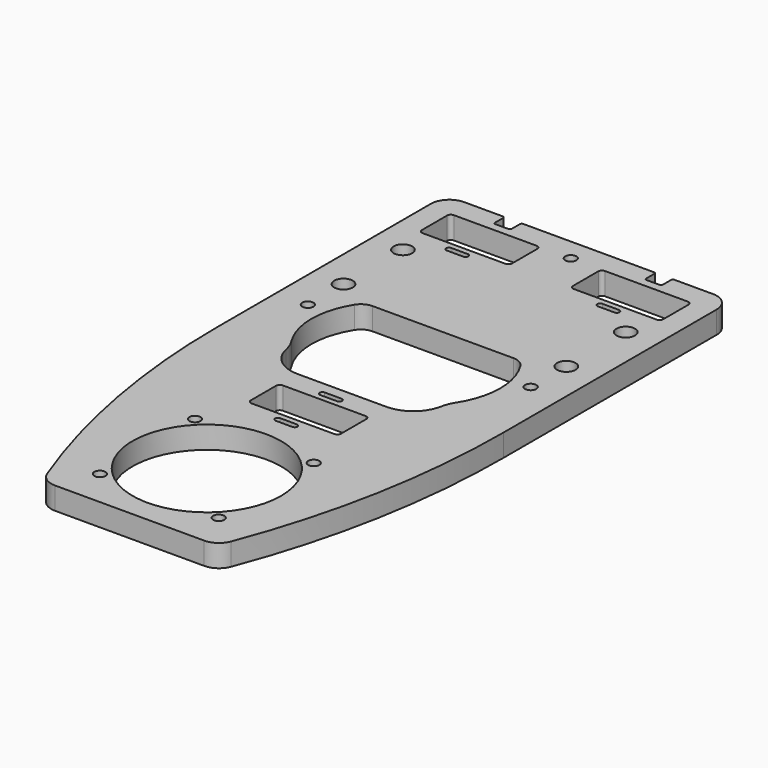
from build123d import *

# Parameters (mm, degrees)
F2_DEPTH = 6
F1_W     = 24.3
F1_H     = 10.5
F1_R     = 2.5
F1_W_2   = 4.5
F1_H_2   = 3.75
F1_R_2   = 1.5
F1_R_3   = 20
F3_DEPTH = 6.001
F4_R     = 1
F5_R     = 0.5
F6_R     = 4
F7_R     = 5
F8_R     = 10


# Not quite as in the source:
# - a feature names something its author has since deleted; it is built from what else it names


with BuildPart() as f2:
    # F0 (on Top) → F2 (new body)
    with BuildSketch(Plane.XY):
        with BuildLine():
            Line((-38.5, 52.75), (-38.5, 41.5))
            Line((-38.5, 41.5), (-38.5, -23.99190475))
            ThreePointArc((-38.5, -23.99190475), (-34.7157474887, -63.5877422109), (-23.5, -101.75))
            Line((-23.5, -101.75), (23.5, -101.75))
            ThreePointArc((23.5, -101.75), (34.7157474887, -63.5877422109), (38.5, -23.99190475))
            Line((38.5, -23.99190475), (38.5, 41.5))
            Line((38.5, 41.5), (38.5, 52.75))
            Line((38.5, 52.75), (-38.5, 52.75))
        make_face()
    extrude(amount=F2_DEPTH)

    # F1 (on Top) → F3 (cut, through all)
    with BuildSketch(Plane.XY):
        with Locations((0, -41.5)):
            Rectangle(F1_W, F1_H)
        with BuildLine():
            ThreePointArc((-2.25, -33.25), (-3, -34), (-2.25, -34.75))
            Line((-2.25, -34.75), (2.25, -34.75))
            ThreePointArc((2.25, -34.75), (3, -34), (2.25, -33.25))
            Line((2.25, -33.25), (-2.25, -33.25))
        make_face()
        with BuildLine():
            ThreePointArc((-21, -21.25), (-18.4168483179, -27.5611508459), (-12.15, -30.25))
            Line((-12.15, -30.25), (12.15, -30.25))
            ThreePointArc((12.15, -30.25), (18.4168483179, -27.5611508459), (21, -21.25))
            ThreePointArc((21, -21.25), (25.387505004, -8.75), (21, 3.75))
            Line((21, 3.75), (-21, 3.75))
            ThreePointArc((-21, 3.75), (-25.387505004, -8.75), (-21, -21.25))
        make_face()
        with Locations((-30, 7.75)):
            Circle(F1_R)
        with Locations((-30, 27.75)):
            Circle(F1_R)
        with Locations((30, 7.75)):
            Circle(F1_R)
        with Locations((30, 27.75)):
            Circle(F1_R)
        with Locations((20.35, 41.5)):
            Rectangle(F1_W, F1_H)
        with BuildLine():
            ThreePointArc((18.1, 34.75), (17.35, 34), (18.1, 33.25))
            Line((18.1, 33.25), (22.6, 33.25))
            ThreePointArc((22.6, 33.25), (23.35, 34), (22.6, 34.75))
            Line((22.6, 34.75), (18.1, 34.75))
        make_face()
        with BuildLine():
            ThreePointArc((-22.6, 34.75), (-23.35, 34), (-22.6, 33.25))
            Line((-22.6, 33.25), (-18.1, 33.25))
            ThreePointArc((-18.1, 33.25), (-17.35, 34), (-18.1, 34.75))
            Line((-18.1, 34.75), (-22.6, 34.75))
        make_face()
        with Locations((-20.35, 41.5)):
            Rectangle(F1_W, F1_H)
        with Locations((-20.35, 50.875)):
            Rectangle(F1_W_2, F1_H_2)
        with Locations((20.35, 50.875)):
            Rectangle(F1_W_2, F1_H_2)
        with Locations((0, 46.75)):
            Circle(F1_R_2)
        with Locations((30, -4.25)):
            Circle(F1_R_2)
        with Locations((-30, -4.25)):
            Circle(F1_R_2)
        with Locations((0, -75.75)):
            Circle(F1_R_3)
        with BuildLine():
            ThreePointArc((-2.25, -48.25), (-3, -49), (-2.25, -49.75))
            Line((-2.25, -49.75), (2.25, -49.75))
            ThreePointArc((2.25, -49.75), (3, -49), (2.25, -48.25))
            Line((2.25, -48.25), (-2.25, -48.25))
        make_face()
        with Locations((16, -59.75)):
            Circle(F1_R_2)
        with Locations((-16, -59.75)):
            Circle(F1_R_2)
        with Locations((16, -91.75)):
            Circle(F1_R_2)
        with Locations((-16, -91.75)):
            Circle(F1_R_2)
    extrude(amount=F3_DEPTH, mode=Mode.SUBTRACT)

    # F4
    f4_edges = [f2.edges().sort_by_distance(p)[0] for p in [
        (12.15, -36.25, 3),
        (-12.15, -36.25, 3),
        (-12.15, -46.75, 3),
        (12.15, -46.75, 3),
        (8.2, 46.75, 3),
        (-32.5, 46.75, 3),
        (-32.5, 36.25, 3),
        (-8.2, 46.75, 3),
        (-8.2, 36.25, 3),
        (32.5, 36.25, 3),
        (8.2, 36.25, 3),
        (32.5, 46.75, 3),
    ]]
    fillet(f4_edges, radius=F4_R)

    # F5
    f5_edges = [f2.edges().sort_by_distance(p)[0] for p in [
        (18.1, 49, 3),
        (22.6, 49, 3),
        (-18.1, 49, 3),
        (-22.6, 49, 3),
        (-22.6, 52.75, 3),
        (-18.1, 52.75, 3),
        (18.1, 52.75, 3),
        (22.6, 52.75, 3),
    ]]
    fillet(f5_edges, radius=F5_R)

    # F6
    f6_edges = [f2.edges().sort_by_distance(p)[0] for p in [
        (-21, 3.75, 3),
        (21, 3.75, 3),
    ]]
    fillet(f6_edges, radius=F6_R)

    # F7
    f7_edges = [f2.edges().sort_by_distance(p)[0] for p in [
        (-23.5, -101.75, 3),
        (23.5, -101.75, 3),
        (-38.5, 52.75, 3),
        (38.5, 52.75, 3),
    ]]
    fillet(f7_edges, radius=F7_R)

    # F8
    f8_edges = [f2.edges().sort_by_distance(p)[0] for p in [
        (-21, -21.25, 3),
        (21, -21.25, 3),
    ]]
    fillet(f8_edges, radius=F8_R)


solid = f2.part
